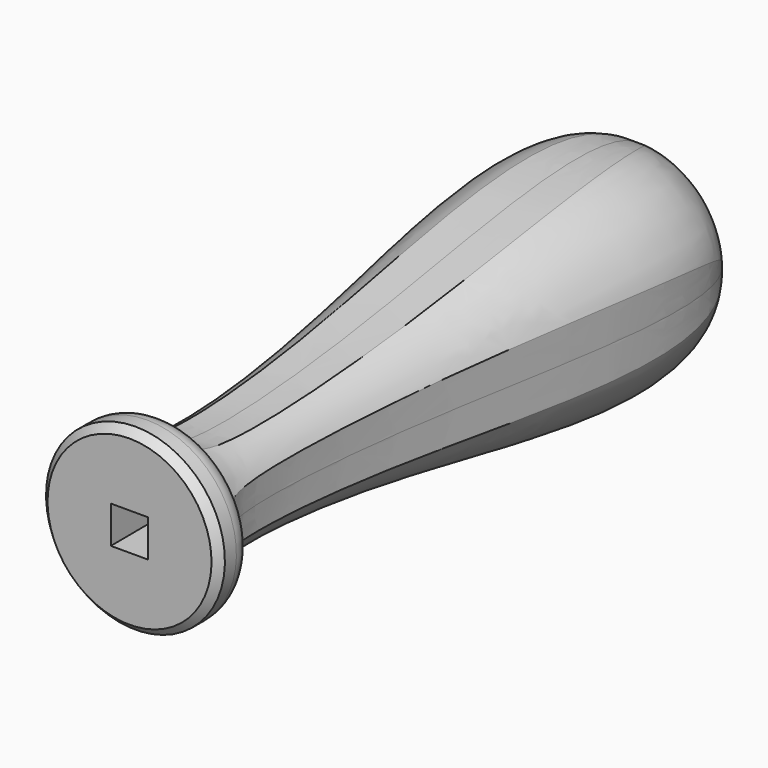
from build123d import *

# Parameters (mm, degrees)
F2_SIZE       = 1
F4_DEPTH      = 5
F4_DEPTH_BACK = 5
F5_COUNT      = 4
F7_R          = 1.5
F8_DEPTH      = 100
F8_DEPTH_BACK = 25
F9_W          = 5
F9_H          = 5
F10_DEPTH     = 35
F10_TAPER     = 2


# Not quite as in the source:
# - the dataset's text gives a spline's control points without its knots; the knots are read off the source's solid


with BuildPart() as f1:
    # F0 (on Right) → F1 (revolve)
    with BuildSketch(Plane.YZ):
        with BuildLine():
            Line((0, 12), (0, 0))
            Line((0, 0), (81.1578258872, 0))
            Line((81.1578258872, 0), (89.6560251713, 0))
            add(Edge.make_bspline(
                [(5.9228962956, 9.1504249722), (6.8900343031, 6.3685388304), (39.5618614962, 7.74400636), (85.7912643516, 19.6263415757), (89.6566016099, 4.5940827585), (89.6560251713, 0)],
                knots=[0, 0, 0, 0, 0.3442049299, 0.770390417, 1, 1, 1, 1], degree=3))
            ThreePointArc((5.9228962956, 9.1504249722), (4.9941231012, 11.1738531363), (2.9266699477, 12))
            Line((2.9266699477, 12), (0, 12))
        make_face()
    revolve(axis=Axis((0, 40.5789129436, 0), (0, -1, 0)))

    # F2
    f2_edges = [f1.edges().sort_by_distance(p)[0] for p in [
        (0, 0, -12),
    ]]
    chamfer(f2_edges, length=F2_SIZE)


with BuildPart() as f4:
    # F3 (on Right) → F4 (new body, two sides)
    with BuildSketch(Plane.YZ) as f4_sk:
        with BuildLine():
            Line((9.9051892757, 31.0736633837), (5.8965189382, 9.1559858993))
            add(Edge.make_bspline(
                [(5.8965189382, 9.1559858993), (5.9472195677, 9.0115264008), (6.0787007332, 8.737855916), (6.4264167356, 8.2752529498), (6.9540357429, 7.8492817721), (7.6695442866, 7.4849318101), (8.477817305, 7.2057885171), (9.3889273865, 6.9862523042), (10.7476798966, 6.7569867165), (12.7180994024, 6.573641292), (15.4916643071, 6.4956271004), (18.6289754692, 6.5476748187), (22.078511792, 6.7198568853), (27.0212738393, 7.0977311992), (32.3663475985, 7.6806858139), (37.8866306932, 8.4350672988), (42.0526870012, 9.0778266944), (46.2117571502, 9.7683310663), (51.7119278945, 10.714634681), (58.4302704603, 11.8739992087), (66.0089075261, 12.9994054756), (72.8627638727, 13.633285281), (77.7556936417, 13.5687704983), (81.0348580655, 13.0706857657), (82.7880556534, 12.5628486358), (83.9981341745, 12.0377737343), (85.0789008782, 11.432460952), (86.1265707678, 10.6022255642), (86.8008379577, 9.8405494507), (87.0694741607, 9.4896582887)],
                knots=[0, 0, 0, 0, 0.0078125, 0.015625, 0.03125, 0.046875, 0.0625, 0.078125, 0.09375, 0.125, 0.15625, 0.1875, 0.21875, 0.25, 0.3125, 0.34375, 0.375, 0.40625, 0.4375, 0.5, 0.5625, 0.625, 0.6875, 0.71875, 0.75, 0.765625, 0.78125, 0.8125, 0.8365570463, 0.8365570463, 0.8365570463, 0.8365570463], degree=3))
            Line((87.0694741607, 9.4896582887), (93.1284055114, 31.0736633837))
            Line((93.1284055114, 31.0736633837), (9.9051892757, 31.0736633837))
        make_face()
    extrude(amount=F4_DEPTH)
    extrude(f4_sk.sketch, amount=-F4_DEPTH_BACK)


with BuildPart() as f5_1:
    # F5: instance of F4
    add(f4.part.rotate(Axis((0, 0, 0), (0, -1, 0)), 1 * 360 / F5_COUNT))


with BuildPart() as f5_2:
    # F5: instance of F4
    add(f4.part.rotate(Axis((0, 0, 0), (0, -1, 0)), 2 * 360 / F5_COUNT))


with BuildPart() as f5_3:
    # F5: instance of F4
    add(f4.part.rotate(Axis((0, 0, 0), (0, -1, 0)), 3 * 360 / F5_COUNT))


with BuildPart() as f1_1:
    add(f1.part)

    # F6: cut F4, F5_1, F5_2, F5_3
    add(f4.part, mode=Mode.SUBTRACT)
    add(f5_1.part, mode=Mode.SUBTRACT)
    add(f5_2.part, mode=Mode.SUBTRACT)
    add(f5_3.part, mode=Mode.SUBTRACT)

    # F7 (on Front) → F8 (cut, two sides)
    with BuildSketch(Plane.XZ) as f8_sk:
        Circle(F7_R)
    extrude(amount=-F8_DEPTH, mode=Mode.SUBTRACT)
    extrude(f8_sk.sketch, amount=F8_DEPTH_BACK, mode=Mode.SUBTRACT)

    # F9 (on Front) → F10 (cut)
    with BuildSketch(Plane.XZ):
        Rectangle(F9_W, F9_H)
    extrude(amount=-F10_DEPTH, taper=F10_TAPER, mode=Mode.SUBTRACT)


solid = f1_1.part
